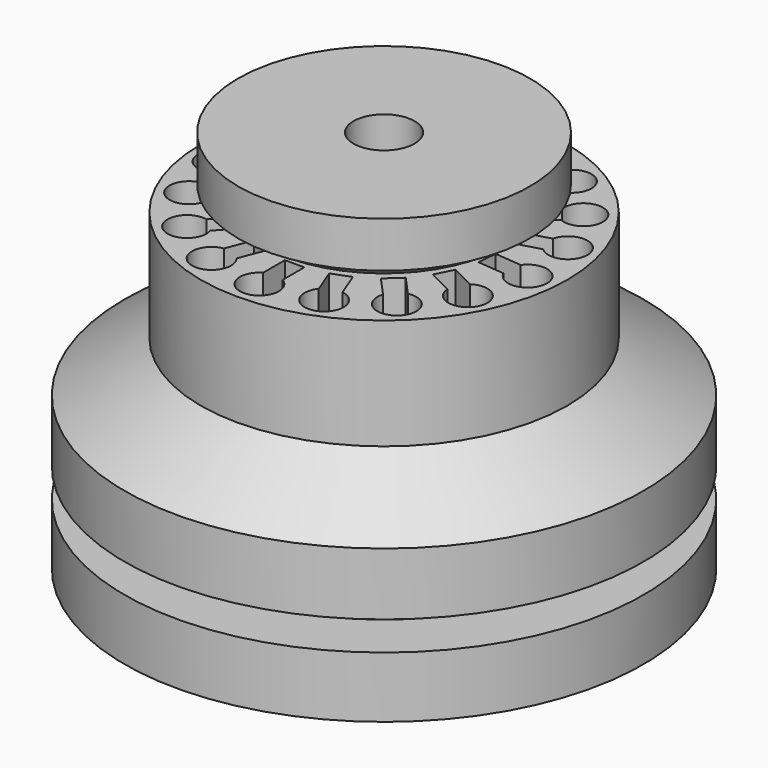
from build123d import *

# Parameters (mm, degrees)
F6_DEPTH        = 19.2430383168
F6_COPIES_COUNT = 17


# Not quite as in the source:
# - a pattern or mirror of a feature is missing from the dataset's text; its kind, count and spacing are read off the source's solid


with BuildPart() as f1:
    # F0 (on Front) → F1 (revolve)
    with BuildSketch(Plane.XZ):
        with BuildLine():
            Line((-17, 4), (-17, 0))
            Line((-17, 0), (-2, 0))
            Line((-2, 0), (-2, 3.5))
            Line((-2, 3.5), (0, 3.5))
            Line((0, 3.5), (0, 5.9224911965))
            Line((0, 5.9224911965), (-2, 5.9224911965))
            Line((-2, 5.9224911965), (-2, 15.4224911965))
            Line((-2, 15.4224911965), (-6.4331775014, 15.4224911965))
            Line((-6.4331775014, 15.4224911965), (-6.4331775014, 14.9095447085))
            ThreePointArc((-6.4331775014, 14.9095447085), (-8.1512170499, 13.7401775165), (-6.4331775014, 12.5708103245))
            Line((-6.4331775014, 12.5708103245), (-6.4331775014, 9.169367192))
            ThreePointArc((-6.4331775014, 9.169367192), (-8.1512170499, 8), (-6.4331775014, 6.830632808))
            Line((-6.4331775014, 6.830632808), (-6.4331775014, 5.6004409318))
            Line((-6.4331775014, 5.6004409318), (-6.4331775014, 4))
            Line((-6.4331775014, 4), (-9.8803927539, 4))
            Line((-9.8803927539, 4), (-10.1592070531, 4))
            ThreePointArc((-10.1592070531, 4), (-11.7589752998, 5.510401574), (-13.3587435466, 4))
            Line((-13.3587435466, 4), (-13.8803896842, 4))
            Line((-13.8803896842, 4), (-17, 4))
        make_face()
    revolve(axis=Axis((0, 0, 4.7112455983), (0, 0, 1)))


with BuildPart() as f2:
    # F0 (on Front) → F2 (revolve)
    with BuildSketch(Plane.XZ):
        Polygon((-17, 5.910401574), (-9.0166758746, 5.910401574), (-8.1612170499, 6.8779131398), (-8.1612170499, 17.9957018993), (-5.968128451, 17.9957018993), (-5.968128451, 20.5524398908), (-12.0092060775, 20.5524398908), (-12.0092060775, 13.2931303233), (-17, 9.9999984652), align=None)
    revolve(axis=Axis((0, 0, 4.7112455983), (0, 0, 1)))

    # F5 (on offset) → F6 (cut, through all)
    with BuildSketch(Plane(origin=(0, 0, 5.910401574), x_dir=(1, 0, 0), z_dir=(0, 0, -1))):
        with BuildLine():
            Line((-0.6377233076, 7.3202499188), (0.6377233076, 7.3202499188))
            Line((0.6377233076, 7.3202499188), (0.6377233076, 9.0992732536))
            ThreePointArc((0.6377233076, 9.0992732536), (0, 11.4803937065), (-0.6377233076, 9.0992732536))
            Line((-0.6377233076, 9.0992732536), (-0.6377233076, 7.3202499188))
        make_face()
    f6 = extrude(amount=-F6_DEPTH, mode=Mode.SUBTRACT)

    # F6_copies: F6 ×17 about axis
    f6_copies_axis = Axis((0, 0, 0), (0, 0, 1))
    for i in range(1, F6_COPIES_COUNT):
        add(f6.rotate(f6_copies_axis, i * 360 / F6_COPIES_COUNT), mode=Mode.SUBTRACT)


with BuildPart() as f3:
    # F0 (on Front) → F3 (revolve)
    with BuildSketch(Plane.XZ):
        with BuildLine():
            Line((-5.568128451, 22.1524398908), (-5.568128451, 16.1224911965))
            Line((-5.568128451, 16.1224911965), (-2, 16.1224911965))
            Line((-2, 16.1224911965), (-2, 25.1524398908))
            Line((-2, 25.1524398908), (-9.568128451, 25.1524398908))
            Line((-9.568128451, 25.1524398908), (-9.568128451, 22.1524398908))
            Line((-9.568128451, 22.1524398908), (-8.468128451, 22.1524398908))
            ThreePointArc((-8.468128451, 22.1524398908), (-7.268128451, 20.9524398908), (-6.068128451, 22.1524398908))
            Line((-6.068128451, 22.1524398908), (-5.568128451, 22.1524398908))
        make_face()
    revolve(axis=Axis((0, 0, 4.7112455983), (0, 0, 1)))


solid = Compound([f1.part, f2.part, f3.part])
